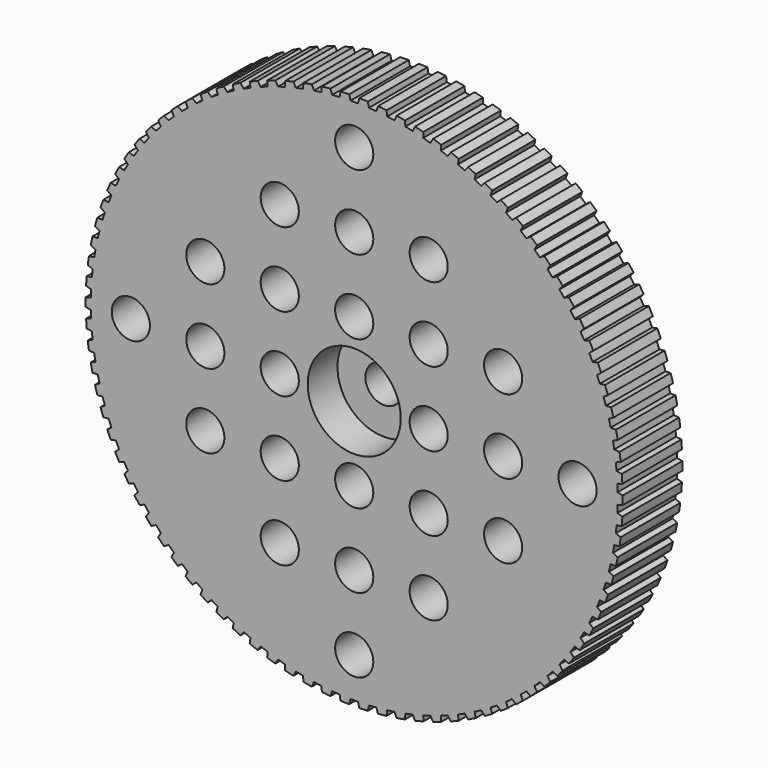
from build123d import *

# Parameters (mm, degrees)
F0_R            = 28.85
F0_R_2          = 2.05
F0_R_3          = 2
F1_DEPTH        = 4
F2_R            = 5
F3_DEPTH        = 4
F5_DEPTH        = 25.4
F5_COPIES_COUNT = 90
F6_R            = 5
F6_R_2          = 2
F7_DEPTH        = 8


# Not quite as in the source:
# - a pattern or mirror of a feature is missing from the dataset's text; its kind, count and spacing are read off the source's solid


with BuildPart() as f1:
    # F0 (on Front) → F1 (new body, symmetric)
    with BuildSketch(Plane.XZ):
        Circle(F0_R)
        with Locations((-8, -16)):
            Circle(F0_R_2, mode=Mode.SUBTRACT)
        with Locations((-16, -8)):
            Circle(F0_R_2, mode=Mode.SUBTRACT)
        with Locations((-8, -8)):
            Circle(F0_R_2, mode=Mode.SUBTRACT)
        with Locations((0, -24)):
            Circle(F0_R_2, mode=Mode.SUBTRACT)
        with Locations((0, -16)):
            Circle(F0_R_2, mode=Mode.SUBTRACT)
        with Locations((8, -16)):
            Circle(F0_R_2, mode=Mode.SUBTRACT)
        with Locations((0, -8)):
            Circle(F0_R_2, mode=Mode.SUBTRACT)
        with Locations((8, -8)):
            Circle(F0_R_2, mode=Mode.SUBTRACT)
        with Locations((16, -8)):
            Circle(F0_R_2, mode=Mode.SUBTRACT)
        with Locations((-24, 0)):
            Circle(F0_R_2, mode=Mode.SUBTRACT)
        with Locations((-16, 0)):
            Circle(F0_R_2, mode=Mode.SUBTRACT)
        with Locations((-16, 8)):
            Circle(F0_R_2, mode=Mode.SUBTRACT)
        with Locations((-8, 0)):
            Circle(F0_R_2, mode=Mode.SUBTRACT)
        with Locations((-8, 8)):
            Circle(F0_R_2, mode=Mode.SUBTRACT)
        with Locations((-8, 16)):
            Circle(F0_R_2, mode=Mode.SUBTRACT)
        Circle(F0_R_3, mode=Mode.SUBTRACT)
        with Locations((8, 0)):
            Circle(F0_R_2, mode=Mode.SUBTRACT)
        with Locations((0, 8)):
            Circle(F0_R_2, mode=Mode.SUBTRACT)
        with Locations((8, 8)):
            Circle(F0_R_2, mode=Mode.SUBTRACT)
        with Locations((16, 0)):
            Circle(F0_R_2, mode=Mode.SUBTRACT)
        with Locations((24, 0)):
            Circle(F0_R_2, mode=Mode.SUBTRACT)
        with Locations((16, 8)):
            Circle(F0_R_2, mode=Mode.SUBTRACT)
        with Locations((0, 16)):
            Circle(F0_R_2, mode=Mode.SUBTRACT)
        with Locations((8, 16)):
            Circle(F0_R_2, mode=Mode.SUBTRACT)
        with Locations((0, 24)):
            Circle(F0_R_2, mode=Mode.SUBTRACT)
    extrude(amount=F1_DEPTH, both=True)

    # F2 (on face) → F3 (cut)
    with BuildSketch(Plane.XZ.offset(4)):
        Circle(F2_R)
    extrude(amount=-F3_DEPTH, mode=Mode.SUBTRACT)

    # F4 (on face) → F5 (cut)
    with BuildSketch(Plane.XZ.offset(4)):
        with BuildLine():
            Line((1.0813484402, 30.84), (-1.0813484402, 30.84))
            Line((-1.0813484402, 30.84), (-0.4, 28.2971730037))
            ThreePointArc((-0.4, 28.2971730037), (0, 28.3), (0.4, 28.2971730037))
            Line((0.4, 28.2971730037), (1.0813484402, 30.84))
        make_face()
    f5 = extrude(amount=-F5_DEPTH, mode=Mode.SUBTRACT)

    # F5_copies: F5 ×90 about axis
    f5_copies_axis = Axis((0, 0, 0), (0, 1, 0))
    for i in range(1, F5_COPIES_COUNT):
        add(f5.rotate(f5_copies_axis, i * 360 / F5_COPIES_COUNT), mode=Mode.SUBTRACT)

    # F6 (on face) → F7 (join)
    with BuildSketch(Plane(origin=(0, 4, 0), x_dir=(-1, 0, 0), z_dir=(0, 1, 0))):
        Circle(F6_R)
        Circle(F6_R_2, mode=Mode.SUBTRACT)
    extrude(amount=F7_DEPTH)


solid = f1.part
